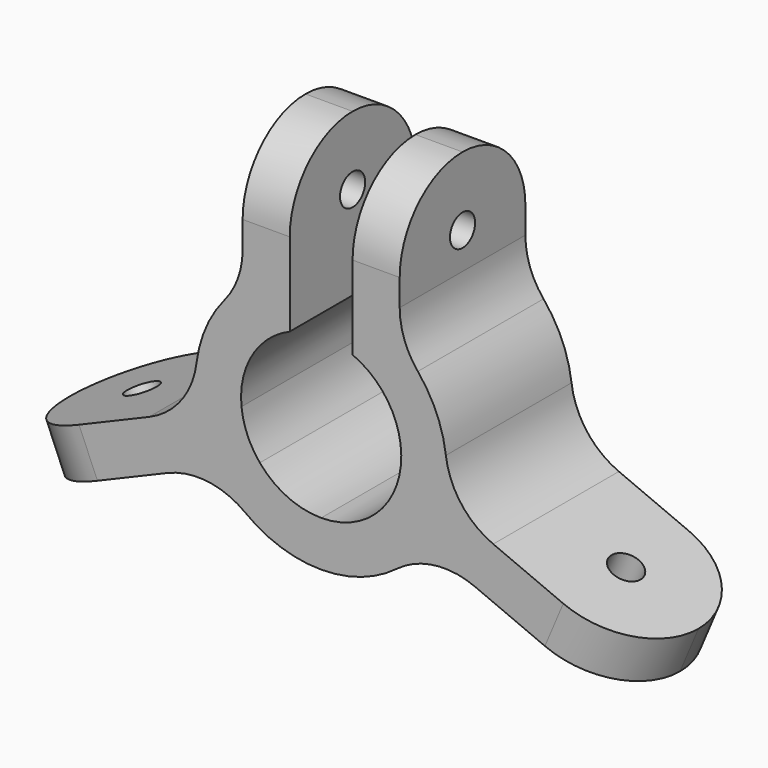
from build123d import *

# Parameters (mm, degrees)
F1_DEPTH = 5
F2_R     = 1
F3_DEPTH = 25
F4_R     = 1
F5_DEPTH = 25
F6_R     = 4.99999
F7_R     = 5


# Not quite as in the source:
# - a fillet or chamfer is up to 0.001 mm smaller than in the source, because OpenCascade refuses the exact size
# - a feature names something its author has since deleted; it is built from what else it names


with BuildPart() as f1:
    # F0 (on Front) → F1 (new body, symmetric)
    with BuildSketch(Plane.XZ):
        with BuildLine():
            ThreePointArc((3.9053168747, -3.2800152603), (2.1542889978, -4.62266578), (0, -5.1))
            Line((0, -5.1), (0, -8))
            ThreePointArc((0, -8), (3.7724872299, -7.0546679653), (6.6534112025, -4.4420850251))
            Line((6.6534112025, -4.4420850251), (3.9053168747, -3.2800152603))
        make_face()
        with BuildLine():
            ThreePointArc((5.0737374807, -0.5169022898), (4.6972920498, -1.9863150301), (3.9053168747, -3.2800152603))
            Line((3.9053168747, -3.2800152603), (6.6534112025, -4.4420850251))
            ThreePointArc((6.6534112025, -4.4420850251), (7.3683012546, -3.1157882825), (7.8218318085, -1.6789720546))
            Line((7.8218318085, -1.6789720546), (5.0737374807, -0.5169022898))
        make_face()
        with BuildLine():
            ThreePointArc((2, 4.6914816423), (4.392181267, 2.5920539573), (5.0737374807, -0.5169022898))
            Line((5.0737374807, -0.5169022898), (7.8218318085, -1.6789720546))
            ThreePointArc((7.8218318085, -1.6789720546), (7.5363895919, 2.683809218), (5, 6.2449979984))
            ThreePointArc((5, 6.2449979984), (3.5795567819, 7.1544932207), (2, 7.7459666924))
            Line((2, 7.7459666924), (2, 4.6914816423))
        make_face()
        with BuildLine():
            ThreePointArc((7.8218318085, -1.6789720546), (7.3683012546, -3.1157882825), (6.6534112025, -4.4420850251))
            Line((6.6534112025, -4.4420850251), (18.8496842561, -9.5994480802))
            Line((18.8496842561, -9.5994480802), (20.018104862, -6.8363351098))
            Line((20.018104862, -6.8363351098), (7.8218318085, -1.6789720546))
        make_face()
        with BuildLine():
            Line((2, 15), (2, 7.7459666924))
            ThreePointArc((2, 7.7459666924), (3.5795567819, 7.1544932207), (5, 6.2449979984))
            Line((5, 6.2449979984), (5, 15))
            Line((5, 15), (2, 15))
        make_face()
    extrude(amount=F1_DEPTH, both=True)

    # F2 (on face) → F3 (cut)
    with BuildSketch(Plane(origin=(0.584210303, 0, 1.3815564852), x_dir=(0.9210376568, 0, -0.3894735353), z_dir=(0.3894735353, 0, 0.9210376568))):
        with Locations((16.1, 0)):
            Circle(F2_R)
    extrude(amount=-F3_DEPTH, mode=Mode.SUBTRACT)

    # F4 (on face) → F5 (cut)
    with BuildSketch(Plane.YZ.offset(5)):
        with Locations((0, 10.6224989992)):
            Circle(F4_R)
    extrude(amount=-F5_DEPTH, mode=Mode.SUBTRACT)

    # F6 (radius 5 in the source; OpenCascade refuses exactly that, so slightly less here)
    f6_edges = [f1.edges().sort_by_distance(p)[0] for p in [
        (19.433895, 5, -8.217892),
        (19.433895, -5, -8.217892),
        (3.5, -5, 15),
        (3.5, 5, 15),
    ]]
    fillet(f6_edges, radius=F6_R)

    # F7
    f7_edges = [f1.edges().sort_by_distance(p)[0] for p in [
        (5, 0, 6.244998),
        (7.821832, 0, -1.678972),
        (6.653411, 0, -4.442085),
    ]]
    fillet(f7_edges, radius=F7_R)

    # F8: F1 across plane


with BuildPart() as f1_1:
    add(f1.part)
    add(f1.part.mirror(Plane.YZ))


solid = f1_1.part
